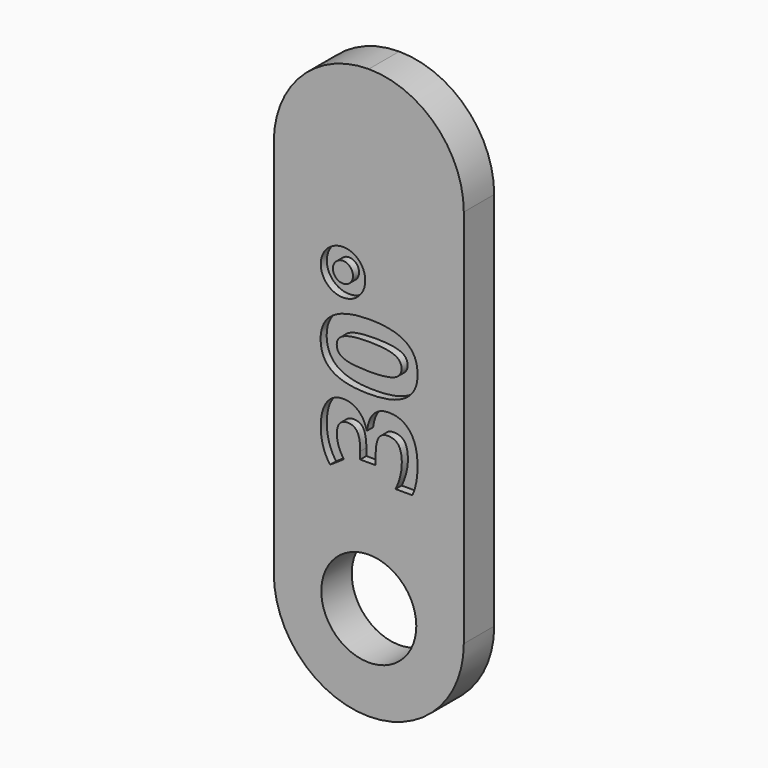
from build123d import *

# Parameters (mm, degrees)
F0_W         = 12.7
F0_H         = 38.1
F0_R         = 3.175
F1_DEPTH     = 2.54
F2_R         = 6.34999
F3_TEXT_SIZE = 8.8194444444
F4_DEPTH     = 0.508


# Not quite as in the source:
# - a fillet or chamfer is up to 0.001 mm smaller than in the source, because OpenCascade refuses the exact size
# - Text() gives the source's letters only with a copy of the font that has no kerning and outlines rounded to 1/6400 em; it was checked with that copy


with BuildPart() as f1:
    # F0 (on Front) → F1 (new body)
    with BuildSketch(Plane.XZ):
        with Locations((6.35, 19.05)):
            Rectangle(F0_W, F0_H)
        with Locations((6.35, 6.35)):
            Circle(F0_R, mode=Mode.SUBTRACT)
    extrude(amount=F1_DEPTH)

    # F2 (radius 6.35 in the source; OpenCascade refuses exactly that, so slightly less here)
    f2_edges = [f1.edges().sort_by_distance(p)[0] for p in [
        (12.7, -1.27, 0),
        (0, -1.27, 0),
        (12.7, -1.27, 38.1),
        (0, -1.27, 38.1),
    ]]
    fillet(f2_edges, radius=F2_R)

    # F3 (on face) → F4 (cut)
    with BuildSketch(Plane.XZ.offset(2.54)):
        with Locations(Location((9.525, 13.6294867622), (0, 0, 90))):
            Text('30°', F3_TEXT_SIZE, font='Open Sans', font_style=FontStyle.BOLD, text_align=(TextAlign.LEFT, TextAlign.BOTTOM))
    extrude(amount=-F4_DEPTH, mode=Mode.SUBTRACT)


solid = f1.part
